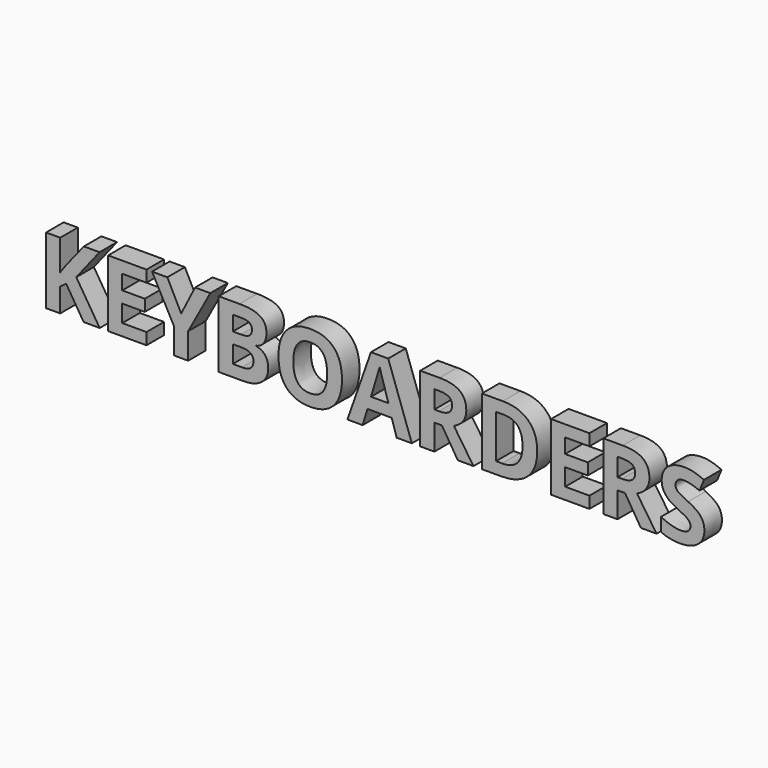
from build123d import *

# Parameters (mm, degrees)
F0_TEXT_SIZE = 108.0417927975
F1_DEPTH     = 25.4


# Not quite as in the source:
# - Text() gives the source's letters only with a copy of the font that has no kerning and outlines rounded to 1/6400 em; it was checked with that copy


with BuildPart() as f1:
    # F0 (on Front) → F1 (new body)
    with BuildSketch(Plane.XZ):
        with Locations((-377.9127150774, -35.7414004393)):
            Text('KEYBOARDERS', F0_TEXT_SIZE, font='Open Sans', font_style=FontStyle.BOLD, text_align=(TextAlign.LEFT, TextAlign.BOTTOM))
    extrude(amount=F1_DEPTH)


solid = f1.part
